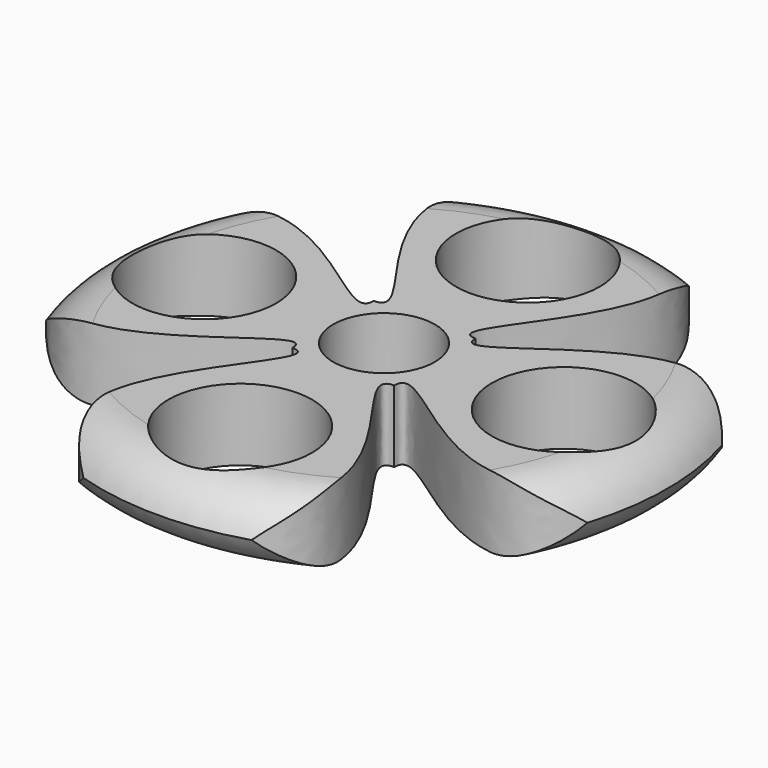
from build123d import *

# Parameters (mm, degrees)
F0_R         = 6.35
F0_R_2       = 4.4901280605
F1_DEPTH     = 6.35
F2_T2_ANGLE  = 86.2531855828
F2_T4_ANGLE  = 86.2531855828
F2_T6_ANGLE  = 86.2531855828
F2_T8_ANGLE  = 86.2531855828
F2_T10_ANGLE = 86.2531855828
F2_T12_ANGLE = 86.2531855828
F2_T14_ANGLE = 86.2531855828
F2_T16_ANGLE = 86.2531855828


# Not quite as in the source:
# - a fillet or chamfer that OpenCascade refuses, or shapes differently, is made with other operations: its cross-section is extruded or revolved along the edge and cut away or added


with BuildPart() as f1:
    # F0 (on Top) → F1 (new body)
    with BuildSketch(Plane.XY):
        with BuildLine():
            add(Edge.make_bspline(
                [(4.4901280605, 4.4901280605), (0, 4.4901280605), (17.9605122421, 17.9605122421), (6.35, 24.5934442484)],
                knots=[0, 0, 0, 0, 20.1891665351, 20.1891665351, 20.1891665351, 20.1891665351], degree=3))
            ThreePointArc((6.35, 24.5934442484), (0, 25.4), (-6.35, 24.5934442484))
            add(Edge.make_bspline(
                [(-4.4901280605, 4.4901280605), (0, 4.4901280605), (-17.9605122421, 17.9605122421), (-6.35, 24.5934442484)],
                knots=[0, 0, 0, 0, 20.1891665351, 20.1891665351, 20.1891665351, 20.1891665351], degree=3))
            add(Edge.make_bspline(
                [(-4.4901280605, 4.4901280605), (-4.4901280605, 0), (-17.9605122421, 17.9605122421), (-24.5934442484, 6.35)],
                knots=[0, 0, 0, 0, 20.1891665351, 20.1891665351, 20.1891665351, 20.1891665351], degree=3))
            ThreePointArc((-24.5934442484, 6.35), (-25.4, 0), (-24.5934442484, -6.35))
            add(Edge.make_bspline(
                [(-4.4901280605, -4.4901280605), (-4.4901280605, 0), (-17.9605122421, -17.9605122421), (-24.5934442484, -6.35)],
                knots=[0, 0, 0, 0, 20.1891665351, 20.1891665351, 20.1891665351, 20.1891665351], degree=3))
            add(Edge.make_bspline(
                [(-4.4901280605, -4.4901280605), (0, -4.4901280605), (-17.9605122421, -17.9605122421), (-6.35, -24.5934442484)],
                knots=[0, 0, 0, 0, 20.1891665351, 20.1891665351, 20.1891665351, 20.1891665351], degree=3))
            ThreePointArc((-6.35, -24.5934442484), (0, -25.4), (6.35, -24.5934442484))
            add(Edge.make_bspline(
                [(4.4901280605, -4.4901280605), (0, -4.4901280605), (17.9605122421, -17.9605122421), (6.35, -24.5934442484)],
                knots=[0, 0, 0, 0, 20.1891665351, 20.1891665351, 20.1891665351, 20.1891665351], degree=3))
            add(Edge.make_bspline(
                [(4.4901280605, -4.4901280605), (4.4901280605, 0), (17.9605122421, -17.9605122421), (24.5934442484, -6.35)],
                knots=[0, 0, 0, 0, 20.1891665351, 20.1891665351, 20.1891665351, 20.1891665351], degree=3))
            ThreePointArc((24.5934442484, -6.35), (25.4, 0), (24.5934442484, 6.35))
            add(Edge.make_bspline(
                [(4.4901280605, 4.4901280605), (4.4901280605, 0), (17.9605122421, 17.9605122421), (24.5934442484, 6.35)],
                knots=[0, 0, 0, 0, 20.1891665351, 20.1891665351, 20.1891665351, 20.1891665351], degree=3))
        make_face()
        with Locations((-15.875, 0)):
            Circle(F0_R, mode=Mode.SUBTRACT)
        with Locations((0, -15.875)):
            Circle(F0_R, mode=Mode.SUBTRACT)
        Circle(F0_R_2, mode=Mode.SUBTRACT)
        with Locations((15.875, 0)):
            Circle(F0_R, mode=Mode.SUBTRACT)
        with Locations((0, 15.875)):
            Circle(F0_R, mode=Mode.SUBTRACT)
    extrude(amount=F1_DEPTH)

    # F2: fillet of radius 5.08 on 8 edges, made by hand

    # F2_s1 → F2_t2 (revolve, cut)
    with BuildSketch(Plane(origin=(0, 0, 0), x_dir=(0, 0, 1), z_dir=(0.7298450689, -0.6836125916, 0))):
        with BuildLine():
            ThreePointArc((1.27, -25.4), (4.8621024484, -23.9121024484), (6.35, -20.32))
            Line((6.35, -20.32), (6.35, -25.4))
            Line((6.35, -25.4), (1.27, -25.4))
        make_face()
    revolve(axis=Axis((0, 0, 6.35), (0, 0, 1)), revolution_arc=F2_T2_ANGLE, mode=Mode.SUBTRACT)

    # F2_s3 → F2_t4 (revolve, cut)
    with BuildSketch(Plane(origin=(0, 0, 0), x_dir=(0, 0, 1), z_dir=(0.7298450689, -0.6836125916, 0))):
        with BuildLine():
            ThreePointArc((5.08, -25.4), (1.4878975516, -23.9121024484), (0, -20.32))
            Line((0, -20.32), (0, -25.4))
            Line((0, -25.4), (5.08, -25.4))
        make_face()
    revolve(axis=Axis((0, 0, 0), (0, 0, 1)), revolution_arc=F2_T4_ANGLE, mode=Mode.SUBTRACT)

    # F2_s5 → F2_t6 (revolve, cut)
    with BuildSketch(Plane(origin=(0, 0, 0), x_dir=(0, 0, 1), z_dir=(-0.6836125916, -0.7298450689, 0))):
        with BuildLine():
            ThreePointArc((1.27, -25.4), (4.8621024484, -23.9121024484), (6.35, -20.32))
            Line((6.35, -20.32), (6.35, -25.4))
            Line((6.35, -25.4), (1.27, -25.4))
        make_face()
    revolve(axis=Axis((0, 0, 6.35), (0, 0, 1)), revolution_arc=F2_T6_ANGLE, mode=Mode.SUBTRACT)

    # F2_s7 → F2_t8 (revolve, cut)
    with BuildSketch(Plane(origin=(0, 0, 0), x_dir=(0, 0, 1), z_dir=(-0.6836125916, -0.7298450689, 0))):
        with BuildLine():
            ThreePointArc((5.08, -25.4), (1.4878975516, -23.9121024484), (0, -20.32))
            Line((0, -20.32), (0, -25.4))
            Line((0, -25.4), (5.08, -25.4))
        make_face()
    revolve(axis=Axis((0, 0, 0), (0, 0, 1)), revolution_arc=F2_T8_ANGLE, mode=Mode.SUBTRACT)

    # F2_s9 → F2_t10 (revolve, cut)
    with BuildSketch(Plane(origin=(0, 0, 0), x_dir=(0, 0, 1), z_dir=(-0.7298450689, 0.6836125916, 0))):
        with BuildLine():
            ThreePointArc((1.27, -25.4), (4.8621024484, -23.9121024484), (6.35, -20.32))
            Line((6.35, -20.32), (6.35, -25.4))
            Line((6.35, -25.4), (1.27, -25.4))
        make_face()
    revolve(axis=Axis((0, 0, 6.35), (0, 0, 1)), revolution_arc=F2_T10_ANGLE, mode=Mode.SUBTRACT)

    # F2_s11 → F2_t12 (revolve, cut)
    with BuildSketch(Plane(origin=(0, 0, 0), x_dir=(0, 0, 1), z_dir=(-0.7298450689, 0.6836125916, 0))):
        with BuildLine():
            ThreePointArc((5.08, -25.4), (1.4878975516, -23.9121024484), (0, -20.32))
            Line((0, -20.32), (0, -25.4))
            Line((0, -25.4), (5.08, -25.4))
        make_face()
    revolve(axis=Axis((0, 0, 0), (0, 0, 1)), revolution_arc=F2_T12_ANGLE, mode=Mode.SUBTRACT)

    # F2_s13 → F2_t14 (revolve, cut)
    with BuildSketch(Plane(origin=(0, 0, 0), x_dir=(0, 0, 1), z_dir=(0.6836125916, 0.7298450689, 0))):
        with BuildLine():
            ThreePointArc((1.27, -25.4), (4.8621024484, -23.9121024484), (6.35, -20.32))
            Line((6.35, -20.32), (6.35, -25.4))
            Line((6.35, -25.4), (1.27, -25.4))
        make_face()
    revolve(axis=Axis((0, 0, 6.35), (0, 0, 1)), revolution_arc=F2_T14_ANGLE, mode=Mode.SUBTRACT)

    # F2_s15 → F2_t16 (revolve, cut)
    with BuildSketch(Plane(origin=(0, 0, 0), x_dir=(0, 0, 1), z_dir=(0.6836125916, 0.7298450689, 0))):
        with BuildLine():
            ThreePointArc((5.08, -25.4), (1.4878975516, -23.9121024484), (0, -20.32))
            Line((0, -20.32), (0, -25.4))
            Line((0, -25.4), (5.08, -25.4))
        make_face()
    revolve(axis=Axis((0, 0, 0), (0, 0, 1)), revolution_arc=F2_T16_ANGLE, mode=Mode.SUBTRACT)


solid = f1.part
